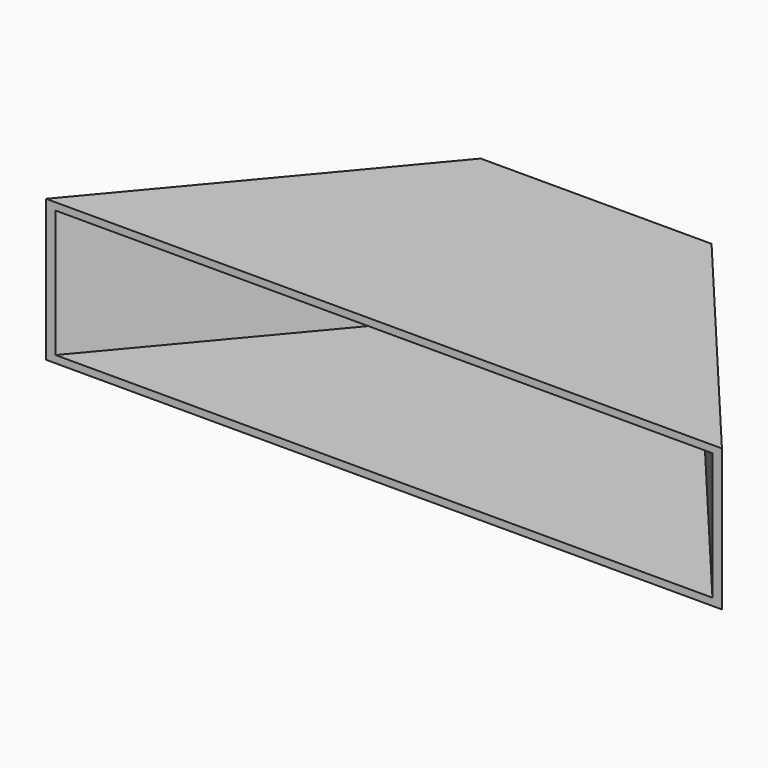
from build123d import *

# Parameters (mm, degrees)
F1_DEPTH = 2
F3_DEPTH = 35
F5_DEPTH = 2


# Not quite as in the source:
# - a feature names something its author has since deleted; it is built from what else it names


with BuildPart() as f1:
    # F0 (on Top) → F1 (new body)
    with BuildSketch(Plane.XY):
        Polygon((-31.75, 72.9657332071), (-92.9755198226, 0), (92.9755198226, 0), (31.75, 72.9657332071), align=None)
    extrude(amount=F1_DEPTH)

    # F2 (on face) → F3 (join)
    with BuildSketch(Plane.XY.offset(2)):
        Polygon((30.8173846837, 70.9657332071), (90.364705244, 0), (92.9755198226, 0), (31.75, 72.9657332071), (-31.75, 72.9657332071), (-92.9755198226, 0), (-90.364705244, 0), (-30.8173846837, 70.9657332071), align=None)
    extrude(amount=F3_DEPTH)

    # F4 (on face) → F5 (join)
    with BuildSketch(Plane.XY.offset(37)):
        Polygon((-31.75, 72.9657332071), (-92.9755198226, 0), (92.9755198226, 0), (31.75, 72.9657332071), align=None)
    extrude(amount=F5_DEPTH)


solid = f1.part
